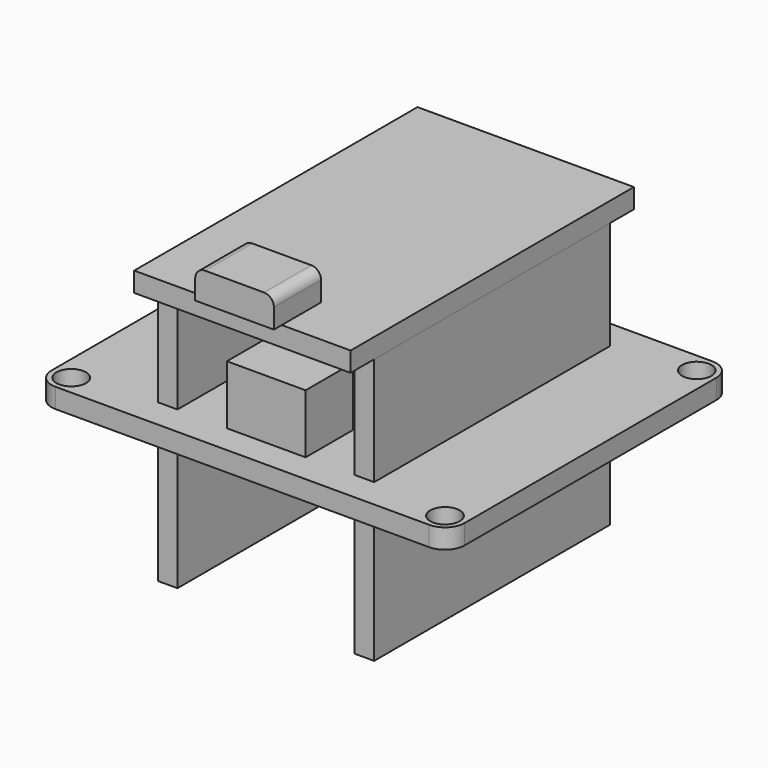
from build123d import *

# Parameters (mm, degrees)
F0_W      = 42
F0_H      = 36
F1_DEPTH  = 2
F2_R      = 2
F3_R      = 1.5
F4_DEPTH  = 2
F5_W      = 2
F5_H      = 30
F6_DEPTH  = 14
F7_W      = 2
F7_H      = 30
F8_DEPTH  = 11
F9_W      = 22
F9_H      = 36
F10_DEPTH = 2
F11_W     = 8
F11_H     = 4.9999979734
F11_H_2   = 1.0000020266
F12_DEPTH = 3
F13_R     = 1
F7_W_2    = 8
F7_H_2    = 6
F14_DEPTH = 6


# Not quite as in the source:
# - a feature names something its author has since deleted; it is built from what else it names


with BuildPart() as f1:
    # F0 (on Top) → F1 (new body)
    with BuildSketch(Plane.XY):
        with Locations((6.745641768, -5.4418604523)):
            Rectangle(F0_W, F0_H)
    extrude(amount=F1_DEPTH)

    # F2
    f2_edges = [f1.edges().sort_by_distance(p)[0] for p in [
        (27.745642, -23.44186, 1),
        (27.745642, 12.55814, 1),
        (-14.254358, -23.44186, 1),
        (-14.254358, 12.55814, 1),
    ]]
    fillet(f2_edges, radius=F2_R)

    # F3 (on face) → F4 (cut)
    with BuildSketch(Plane.XY.offset(2)):
        with Locations((-12.254358232, 10.5581395477)):
            Circle(F3_R)
        with Locations((-12.254358232, -21.4418604523)):
            Circle(F3_R)
        with Locations((25.745641768, -21.4418604523)):
            Circle(F3_R)
        with Locations((25.745641768, 10.5581395477)):
            Circle(F3_R)
    extrude(amount=-F4_DEPTH, mode=Mode.SUBTRACT)

    # F5 (on face) → F6 (join)
    with BuildSketch(Plane(origin=(0, 0, 0), x_dir=(1, 0, 0), z_dir=(0, 0, -1))):
        with Locations((16.7456435263, 5.4418606311)):
            Rectangle(F5_W, F5_H)
        with Locations((-3.2543599904, 5.4418606311)):
            Rectangle(F5_W, F5_H)
    extrude(amount=F6_DEPTH)

    # F7 (on face) → F8 (join)
    with BuildSketch(Plane.XY.offset(2)):
        with Locations((16.7456435263, -5.4418606311)):
            Rectangle(F7_W, F7_H)
        with Locations((-3.2543599904, -5.4418606311)):
            Rectangle(F7_W, F7_H)
    extrude(amount=F8_DEPTH)

    # F9 (on face) → F10 (join)
    with BuildSketch(Plane.XY.offset(13)):
        with Locations((6.7456400096, -5.4360154718)):
            Rectangle(F9_W, F9_H)
    extrude(amount=F10_DEPTH)

    # F11 (on face) → F12 (join)
    with BuildSketch(Plane.XY.offset(15)):
        with Locations((6.7456399985, -20.9360164851)):
            Rectangle(F11_W, F11_H)
        with Locations((6.7456399985, -23.9360164851)):
            Rectangle(F11_W, F11_H_2)
    extrude(amount=F12_DEPTH)

    # F13
    f13_edges = [f1.edges().sort_by_distance(p)[0] for p in [
        (10.74564, -21.436017, 18),
        (2.74564, -21.436017, 18),
    ]]
    fillet(f13_edges, radius=F13_R)

    # F7 (on face) → F14 (join)
    with BuildSketch(Plane.XY.offset(2)):
        with Locations((6.829907462, -17.511118643)):
            Rectangle(F7_W_2, F7_H_2)
    extrude(amount=F14_DEPTH)


with BuildPart() as f15_1:
    # F15: copy of F1
    add(f1.part)


solid = f1.part
